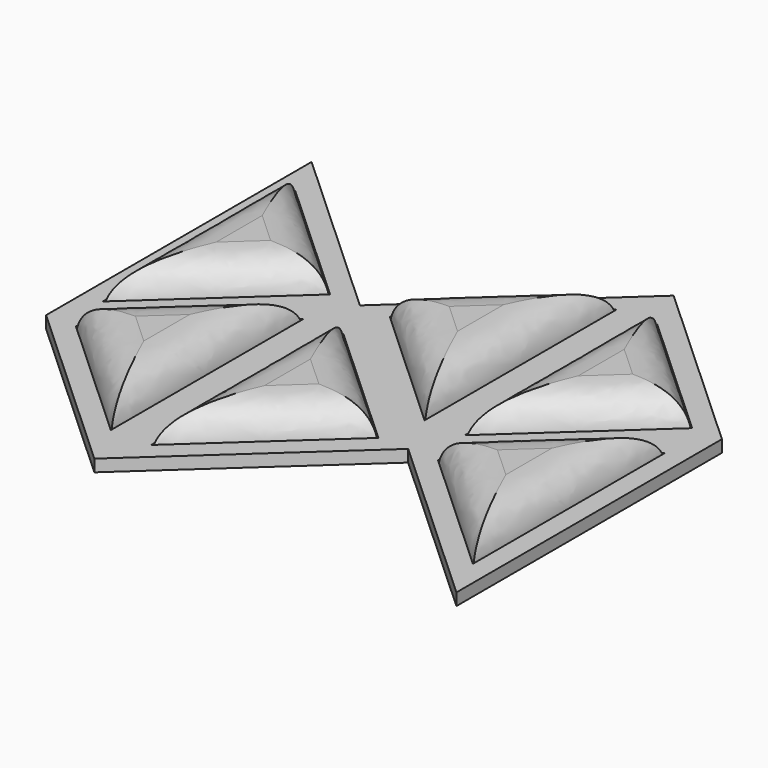
from build123d import *

# Parameters (mm, degrees)
F2_DEPTH      = 20
F3_DEPTH      = 6
F4_T1_DEPTH   = 328.4497108295
F4_T3_DEPTH   = 328.4497153004
F4_T5_DEPTH   = 359.5352990065
F4_2_T1_DEPTH = 219.5352975776
F4_2_T3_DEPTH = 188.4497097722
F4_2_T5_DEPTH = 188.4497097722
F4_3_T1_DEPTH = 219.5352975776
F4_3_T3_DEPTH = 188.4497097722
F4_3_T5_DEPTH = 188.4497097722
F4_4_T1_DEPTH = 188.4497097722
F4_4_T3_DEPTH = 219.5352975776
F4_4_T5_DEPTH = 188.4497097722
F4_5_T1_DEPTH = 188.4497163576
F4_5_T3_DEPTH = 219.5353004354
F4_5_T5_DEPTH = 188.4497163576
F4_6_T1_DEPTH = 188.4497163576
F4_6_T3_DEPTH = 219.5353004354
F4_6_T5_DEPTH = 188.4497163576


# Not quite as in the source:
# - a fillet or chamfer that OpenCascade refuses, or shapes differently, is made with other operations: its cross-section is extruded or revolved along the edge and cut away or added


with BuildPart() as f2:
    # F1 (on Top) → F2 (new body)
    with BuildSketch(Plane.XY):
        Polygon((-86.440576249, -108.7447496522), (-21.2395070962, -48.9771001489), (-86.4405823141, 10.7905493543), align=None)
    extrude(amount=F2_DEPTH)

    # F4: fillet of radius 20 on 3 edges, made by hand

    # F4_s2 → F4_t1 (cut)
    with BuildSketch(Plane(origin=(-189.5971721651, -173.7974159014, 0), x_dir=(0, 0, 1), z_dir=(0.7371541245, 0.6757246456, 0))):
        with BuildLine():
            add(Edge.make_bspline(
                [(0, 21.7516129779), (20, 21.7516129779), (20, 1.7516129779)],
                knots=[0, 0, 0, 1, 1, 1], degree=2, weights=[1, 1, 1]))
            Line((20, 1.7516129779), (20.4, 1.7516129779))
            Line((20.4, 1.7516129779), (20.4, 22.1516129779))
            Line((20.4, 22.1516129779), (0, 22.1516129779))
            Line((0, 22.1516129779), (0, 21.7516129779))
        make_face()
    extrude(amount=F4_T1_DEPTH, mode=Mode.SUBTRACT)

    # F4_s4 → F4_t3 (cut)
    with BuildSketch(Plane(origin=(101.3131705585, -92.8704020259, 0), x_dir=(0, 0, 1), z_dir=(-0.7371541559, 0.6757246114, 0))):
        with BuildLine():
            add(Edge.make_bspline(
                [(0, -50.4557305963), (20, -50.4557305963), (20, -70.4557305963)],
                knots=[0, 0, 0, 1, 1, 1], degree=2, weights=[1, 1, 1]))
            Line((20, -70.4557305963), (20.4, -70.4557305963))
            Line((20.4, -70.4557305963), (20.4, -50.0557305963))
            Line((20.4, -50.0557305963), (0, -50.0557305963))
            Line((0, -50.0557305963), (0, -50.4557305963))
        make_face()
    extrude(amount=F4_T3_DEPTH, mode=Mode.SUBTRACT)

    # F4_s6 → F4_t5 (cut)
    with BuildSketch(Plane.XZ.offset(-130.7905493543)):
        with BuildLine():
            add(Edge.make_bspline(
                [(-86.4405884027, 0), (-86.4405884027, 20), (-66.4405884027, 20)],
                knots=[0, 0, 0, 1, 1, 1], degree=2, weights=[1, 1, 1]))
            Line((-66.4405884027, 20), (-66.4405884027, 20.4))
            Line((-66.4405884027, 20.4), (-86.8405884027, 20.4))
            Line((-86.8405884027, 20.4), (-86.8405884027, 0))
            Line((-86.8405884027, 0), (-86.4405884027, 0))
        make_face()
    extrude(amount=F4_T5_DEPTH, mode=Mode.SUBTRACT)


with BuildPart() as f2b:
    # F1 (on Top) → F2, piece 2 (new body)
    with BuildSketch(Plane.XY):
        Polygon((-16.4405792815, -191.2447485949), (-16.4405792815, -71.7094510173), (-81.641647655, -131.4770998061), align=None)
    extrude(amount=F2_DEPTH)

    # F4#2: fillet of radius 20 on 3 edges, made by hand

    # F4_2_s2 → F4_2_t1 (cut)
    with BuildSketch(Plane.XZ.offset(21.7094510173)):
        with BuildLine():
            add(Edge.make_bspline(
                [(-16.4405792815, 0), (-16.4405792815, 20), (-36.4405792815, 20)],
                knots=[0, 0, 0, 1, 1, 1], degree=2, weights=[1, 1, 1]))
            Line((-36.4405792815, 20), (-16.4405792815, 20))
            Line((-16.4405792815, 20), (-16.4405792815, 0))
        make_face()
    extrude(amount=F4_2_T1_DEPTH, mode=Mode.SUBTRACT)

    # F4_2_s4 → F4_2_t3 (cut)
    with BuildSketch(Plane(origin=(-7.7954669368, -7.1458450244, 0), x_dir=(0, 0, 1), z_dir=(-0.7371541245, -0.6757246456, 0))):
        with BuildLine():
            add(Edge.make_bspline(
                [(0, -41.7516129779), (20, -41.7516129779), (20, -61.7516129779)],
                knots=[0, 0, 0, 1, 1, 1], degree=2, weights=[1, 1, 1]))
            Line((20, -61.7516129779), (20, -41.7516129779))
            Line((20, -41.7516129779), (0, -41.7516129779))
        make_face()
    extrude(amount=F4_2_T3_DEPTH, mode=Mode.SUBTRACT)

    # F4_2_s6 → F4_2_t5 (cut)
    with BuildSketch(Plane(origin=(-15.7309874293, 14.4200724808, 0), x_dir=(0, 0, 1), z_dir=(0.7371541245, -0.6757246456, 0))):
        with BuildLine():
            add(Edge.make_bspline(
                [(0, 152.0861598329), (20, 152.0861598329), (20, 132.0861598329)],
                knots=[0, 0, 0, 1, 1, 1], degree=2, weights=[1, 1, 1]))
            Line((20, 132.0861598329), (20, 152.0861598329))
            Line((20, 152.0861598329), (0, 152.0861598329))
        make_face()
    extrude(amount=F4_2_T5_DEPTH, mode=Mode.SUBTRACT)


with BuildPart() as f2c:
    # F1 (on Top) → F2, piece 3 (new body)
    with BuildSketch(Plane.XY):
        Polygon((3.5594207185, -191.2447485949), (68.7604890919, -131.4770998061), (3.5594207185, -71.7094510173), align=None)
    extrude(amount=F2_DEPTH)

    # F4#3: fillet of radius 20 on 3 edges, made by hand

    # F4_3_s2 → F4_3_t1 (cut)
    with BuildSketch(Plane.XZ.offset(21.7094510173)):
        with BuildLine():
            add(Edge.make_bspline(
                [(3.5594207185, 0), (3.5594207185, 20), (23.5594207185, 20)],
                knots=[0, 0, 0, 1, 1, 1], degree=2, weights=[1, 1, 1]))
            Line((23.5594207185, 20), (3.5594207185, 20))
            Line((3.5594207185, 20), (3.5594207185, 0))
        make_face()
    extrude(amount=F4_3_T1_DEPTH, mode=Mode.SUBTRACT)

    # F4_3_s4 → F4_3_t3 (cut)
    with BuildSketch(Plane(origin=(-130.1850660565, -119.3363161022, 0), x_dir=(0, 0, 1), z_dir=(0.7371541245, 0.6757246456, 0))):
        with BuildLine():
            add(Edge.make_bspline(
                [(0, 143.382043528), (20, 143.382043528), (20, 123.382043528)],
                knots=[0, 0, 0, 1, 1, 1], degree=2, weights=[1, 1, 1]))
            Line((20, 123.382043528), (20, 143.382043528))
            Line((20, 143.382043528), (0, 143.382043528))
        make_face()
    extrude(amount=F4_3_T3_DEPTH, mode=Mode.SUBTRACT)

    # F4_3_s6 → F4_3_t5 (cut)
    with BuildSketch(Plane(origin=(139.7123751071, -128.0696831381, 0), x_dir=(0, 0, 1), z_dir=(-0.7371541245, 0.6757246456, 0))):
        with BuildLine():
            add(Edge.make_bspline(
                [(0, -50.4557292828), (20, -50.4557292828), (20, -70.4557292828)],
                knots=[0, 0, 0, 1, 1, 1], degree=2, weights=[1, 1, 1]))
            Line((20, -70.4557292828), (20, -50.4557292828))
            Line((20, -50.4557292828), (0, -50.4557292828))
        make_face()
    extrude(amount=F4_3_T5_DEPTH, mode=Mode.SUBTRACT)


with BuildPart() as f2d:
    # F1 (on Top) → F2, piece 4 (new body)
    with BuildSketch(Plane.XY):
        Polygon((73.5594165325, -108.7447485949), (73.5594165325, 10.7905489827), (8.3583481591, -48.9770998061), align=None)
    extrude(amount=F2_DEPTH)

    # F4#4: fillet of radius 20 on 3 edges, made by hand

    # F4_4_s2 → F4_4_t1 (cut)
    with BuildSketch(Plane(origin=(-7.9196711923, 7.2596989306, 0), x_dir=(0, 0, 1), z_dir=(0.7371541245, -0.6757246456, 0))):
        with BuildLine():
            add(Edge.make_bspline(
                [(0, 30.4557292828), (20, 30.4557292828), (20, 10.4557292828)],
                knots=[0, 0, 0, 1, 1, 1], degree=2, weights=[1, 1, 1]))
            Line((20, 10.4557292828), (20, 30.4557292828))
            Line((20, 30.4557292828), (0, 30.4557292828))
        make_face()
    extrude(amount=F4_4_T1_DEPTH, mode=Mode.SUBTRACT)

    # F4_4_s4 → F4_4_t3 (cut)
    with BuildSketch(Plane.XZ.offset(-60.7905489827)):
        with BuildLine():
            add(Edge.make_bspline(
                [(73.5594165325, 0), (73.5594165325, 20), (53.5594165325, 20)],
                knots=[0, 0, 0, 1, 1, 1], degree=2, weights=[1, 1, 1]))
            Line((53.5594165325, 20), (73.5594165325, 20))
            Line((73.5594165325, 20), (73.5594165325, 0))
        make_face()
    extrude(amount=F4_4_T3_DEPTH, mode=Mode.SUBTRACT)

    # F4_4_s6 → F4_4_t5 (cut)
    with BuildSketch(Plane(origin=(82.2045288773, 75.3541549756, 0), x_dir=(0, 0, 1), z_dir=(-0.7371541245, -0.6757246456, 0))):
        with BuildLine():
            add(Edge.make_bspline(
                [(0, -41.7516129779), (20, -41.7516129779), (20, -61.7516129779)],
                knots=[0, 0, 0, 1, 1, 1], degree=2, weights=[1, 1, 1]))
            Line((20, -61.7516129779), (20, -41.7516129779))
            Line((20, -41.7516129779), (0, -41.7516129779))
        make_face()
    extrude(amount=F4_4_T5_DEPTH, mode=Mode.SUBTRACT)


with BuildPart() as f2e:
    # F1 (on Top) → F2, piece 5 (new body)
    with BuildSketch(Plane.XY):
        Polygon((158.7604925298, -48.9770998061), (93.5594165325, 10.7905504116), (93.5594165325, -108.7447500238), align=None)
    extrude(amount=F2_DEPTH)

    # F4#5: fillet of radius 20 on 3 edges, made by hand

    # F4_5_s2 → F4_5_t1 (cut)
    with BuildSketch(Plane(origin=(147.5237041838, -135.2300558788, 0), x_dir=(0, 0, 1), z_dir=(-0.7371541559, 0.6757246114, 0))):
        with BuildLine():
            add(Edge.make_bspline(
                [(0, 71.1746994628), (20, 71.1746994628), (20, 51.1746994628)],
                knots=[0, 0, 0, 1, 1, 1], degree=2, weights=[1, 1, 1]))
            Line((20, 51.1746994628), (20, 71.1746994628))
            Line((20, 71.1746994628), (0, 71.1746994628))
        make_face()
    extrude(amount=F4_5_T1_DEPTH, mode=Mode.SUBTRACT)

    # F4_5_s4 → F4_5_t3 (cut)
    with BuildSketch(Plane.XZ.offset(-60.7905504116)):
        with BuildLine():
            add(Edge.make_bspline(
                [(93.5594165325, 0), (93.5594165325, 20), (113.5594165325, 20)],
                knots=[0, 0, 0, 1, 1, 1], degree=2, weights=[1, 1, 1]))
            Line((113.5594165325, 20), (93.5594165325, 20))
            Line((93.5594165325, 20), (93.5594165325, 0))
        make_face()
    extrude(amount=F4_5_T3_DEPTH, mode=Mode.SUBTRACT)

    # F4_5_s6 → F4_5_t5 (cut)
    with BuildSketch(Plane(origin=(-40.1850677636, -36.8363104034, 0), x_dir=(0, 0, 1), z_dir=(0.7371541559, 0.6757246114, 0))):
        with BuildLine():
            add(Edge.make_bspline(
                [(0, 143.3820447904), (20, 143.3820447904), (20, 123.3820447904)],
                knots=[0, 0, 0, 1, 1, 1], degree=2, weights=[1, 1, 1]))
            Line((20, 123.3820447904), (20, 143.3820447904))
            Line((20, 143.3820447904), (0, 143.3820447904))
        make_face()
    extrude(amount=F4_5_T5_DEPTH, mode=Mode.SUBTRACT)


with BuildPart() as f2f:
    # F1 (on Top) → F2, piece 6 (new body)
    with BuildSketch(Plane.XY):
        Polygon((98.3583447212, -131.4770998061), (163.5594207185, -191.2447500238), (163.5594207185, -71.7094495884), align=None)
    extrude(amount=F2_DEPTH)

    # F4#6: fillet of radius 20 on 3 edges, made by hand

    # F4_6_s2 → F4_6_t1 (cut)
    with BuildSketch(Plane(origin=(82.0803274743, -75.2402966853, 0), x_dir=(0, 0, 1), z_dir=(0.7371541559, -0.6757246114, 0))):
        with BuildLine():
            add(Edge.make_bspline(
                [(0, 30.4557362534), (20, 30.4557362534), (20, 10.4557362534)],
                knots=[0, 0, 0, 1, 1, 1], degree=2, weights=[1, 1, 1]))
            Line((20, 10.4557362534), (20, 30.4557362534))
            Line((20, 30.4557362534), (0, 30.4557362534))
        make_face()
    extrude(amount=F4_6_T1_DEPTH, mode=Mode.SUBTRACT)

    # F4_6_s4 → F4_6_t3 (cut)
    with BuildSketch(Plane.XZ.offset(21.7094495884)):
        with BuildLine():
            add(Edge.make_bspline(
                [(163.5594207185, 0), (163.5594207185, 20), (143.5594207185, 20)],
                knots=[0, 0, 0, 1, 1, 1], degree=2, weights=[1, 1, 1]))
            Line((143.5594207185, 20), (163.5594207185, 20))
            Line((163.5594207185, 20), (163.5594207185, 0))
        make_face()
    extrude(amount=F4_6_T3_DEPTH, mode=Mode.SUBTRACT)

    # F4_6_s6 → F4_6_t5 (cut)
    with BuildSketch(Plane(origin=(90.0158597791, 82.514534293, 0), x_dir=(0, 0, 1), z_dir=(-0.7371541559, -0.6757246114, 0))):
        with BuildLine():
            add(Edge.make_bspline(
                [(0, -163.3820447904), (20, -163.3820447904), (20, -183.3820447904)],
                knots=[0, 0, 0, 1, 1, 1], degree=2, weights=[1, 1, 1]))
            Line((20, -183.3820447904), (20, -163.3820447904))
            Line((20, -163.3820447904), (0, -163.3820447904))
        make_face()
    extrude(amount=F4_6_T5_DEPTH, mode=Mode.SUBTRACT)


with BuildPart() as f3:
    # F1 (on Top) → F3 (new body)
    with BuildSketch(Plane.XY):
        Polygon((-6.4405792815, -48.9770998061), (-96.4405834675, 33.5229001939), (-96.4405750956, -131.4770998061), align=None)
        Polygon((-86.4405823141, 10.7905493543), (-21.2395070962, -48.9771001489), (-86.440576249, -108.7447496522), align=None, mode=Mode.SUBTRACT)
        Polygon((-6.4405792815, -213.9770998061), (-6.4405792815, -48.9770998061), (-96.4405750956, -131.4770998061), align=None)
        Polygon((-81.641647655, -131.4770998061), (-16.4405792815, -71.7094510173), (-16.4405792815, -191.2447485949), align=None, mode=Mode.SUBTRACT)
        Polygon((83.5594165325, -131.4770998061), (-6.4405792815, -48.9770998061), (-6.4405792815, -213.9770998061), align=None)
        Polygon((3.5594207185, -71.7094510173), (68.7604890919, -131.4770998061), (3.5594207185, -191.2447485949), align=None, mode=Mode.SUBTRACT)
        Polygon((173.5594207185, -48.9770998061), (83.5594165325, 33.5229001939), (83.5594165325, -131.4770998061), align=None)
        Polygon((93.5594165325, -108.7447500238), (93.5594165325, 10.7905504116), (158.7604925298, -48.9770998061), align=None, mode=Mode.SUBTRACT)
        Polygon((83.5594165325, 33.5229001939), (-6.4405792815, -48.9770998061), (83.5594165325, -131.4770998061), align=None)
        Polygon((8.3583481591, -48.9770998061), (73.5594165325, 10.7905489827), (73.5594165325, -108.7447485949), align=None, mode=Mode.SUBTRACT)
        Polygon((173.5594207185, -48.9770998061), (83.5594165325, -131.4770998061), (173.5594207185, -213.9770998061), align=None)
        Polygon((163.5594207185, -71.7094495884), (163.5594207185, -191.2447500238), (98.3583447212, -131.4770998061), align=None, mode=Mode.SUBTRACT)
    extrude(amount=F3_DEPTH)


solid = Compound([f2.part, f2b.part, f2c.part, f2d.part, f2e.part, f2f.part, f3.part])
